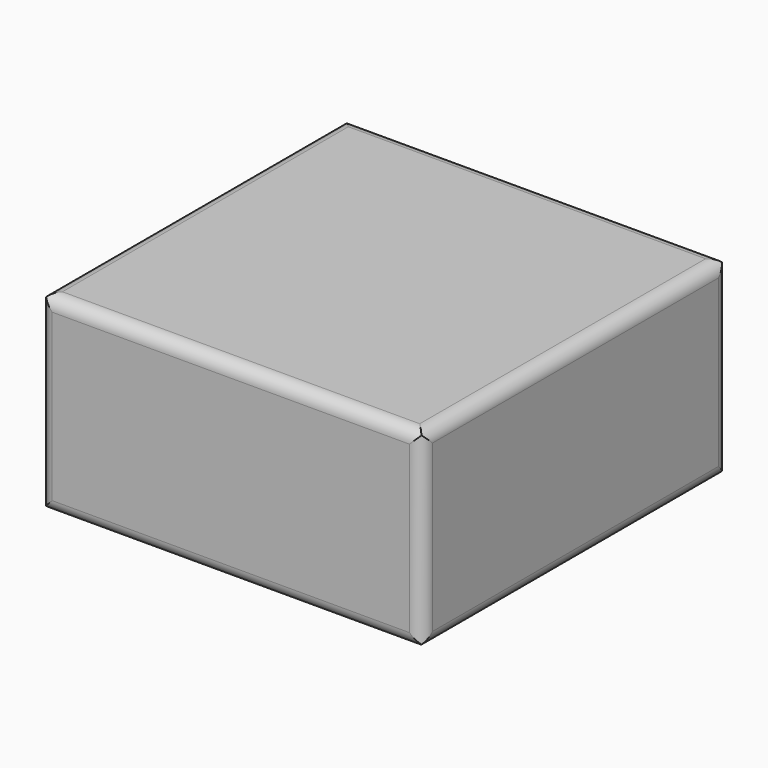
from build123d import *

# Parameters (mm, degrees)
F0_W        = 150
F0_H        = 150
F1_DEPTH    = 75
F2_R        = 5
F3_T1_DEPTH = 170
F3_T3_DEPTH = 100
F4_T1_DEPTH = 170
F4_T3_DEPTH = 100
F5_T1_DEPTH = 165


# Not quite as in the source:
# - a fillet or chamfer that OpenCascade refuses, or shapes differently, is made with other operations: its cross-section is extruded or revolved along the edge and cut away or added


with BuildPart() as f1:
    # F0 (on Top) → F1 (new body)
    with BuildSketch(Plane.XY):
        with Locations((-1.1938624084, 0.1442111853)):
            Rectangle(F0_W, F0_H)
    extrude(amount=F1_DEPTH)

    # F2
    f2_edges = [f1.edges().sort_by_distance(p)[0] for p in [
        (-76.193862, -74.855789, 37.5),
        (73.806138, -74.855789, 37.5),
        (-1.193862, -74.855789, 0),
        (-1.193862, -74.855789, 75),
    ]]
    fillet(f2_edges, radius=F2_R)

    # F3: fillet of radius 5 on 4 edges, made by hand

    # F3_s2 → F3_t1 (cut)
    with BuildSketch(Plane.XZ.offset(-87.6442111853)):
        with BuildLine():
            ThreePointArc((68.8061375916, 0), (72.3416714975, 1.4644660941), (73.8061375916, 5))
            Line((73.8061375916, 5), (73.8061375916, 0))
            Line((73.8061375916, 0), (68.8061375916, 0))
        make_face()
        with BuildLine():
            ThreePointArc((68.8061375916, 75), (72.3416714975, 73.5355339059), (73.8061375916, 70))
            Line((73.8061375916, 70), (73.8061375916, 75))
            Line((73.8061375916, 75), (68.8061375916, 75))
        make_face()
    extrude(amount=F3_T1_DEPTH, mode=Mode.SUBTRACT)

    # F3_s4 → F3_t3 (cut)
    with BuildSketch(Plane.XY.offset(-12.5)):
        with BuildLine():
            ThreePointArc((68.8061375916, 75.1442111853), (72.3416714975, 73.6797450912), (73.8061375916, 70.1442111853))
            Line((73.8061375916, 70.1442111853), (73.8061375916, 75.1442111853))
            Line((73.8061375916, 75.1442111853), (68.8061375916, 75.1442111853))
        make_face()
    extrude(amount=F3_T3_DEPTH, mode=Mode.SUBTRACT)

    # F4: fillet of radius 5 on 4 edges, made by hand

    # F4_s2 → F4_t1 (cut)
    with BuildSketch(Plane.YZ.offset(-88.6938624084)):
        with BuildLine():
            ThreePointArc((70.1442111853, 0), (73.6797450912, 1.4644660941), (75.1442111853, 5))
            Line((75.1442111853, 5), (75.1442111853, 0))
            Line((75.1442111853, 0), (70.1442111853, 0))
        make_face()
        with BuildLine():
            ThreePointArc((75.1442111853, 70), (73.6797450912, 73.5355339059), (70.1442111853, 75))
            Line((70.1442111853, 75), (75.1442111853, 75))
            Line((75.1442111853, 75), (75.1442111853, 70))
        make_face()
    extrude(amount=F4_T1_DEPTH, mode=Mode.SUBTRACT)

    # F4_s4 → F4_t3 (cut)
    with BuildSketch(Plane.XY.offset(-12.5)):
        with BuildLine():
            ThreePointArc((-76.1938624084, 70.1442111853), (-74.7293963143, 73.6797450912), (-71.1938624084, 75.1442111853))
            Line((-71.1938624084, 75.1442111853), (-76.1938624084, 75.1442111853))
            Line((-76.1938624084, 75.1442111853), (-76.1938624084, 70.1442111853))
        make_face()
    extrude(amount=F4_T3_DEPTH, mode=Mode.SUBTRACT)

    # F5: fillet of radius 5 on 4 edges, made by hand

    # F5_s2 → F5_t1 (cut)
    with BuildSketch(Plane.XZ.offset(-82.6442111853)):
        with BuildLine():
            ThreePointArc((-76.1938624084, 5), (-74.7293963143, 1.4644660941), (-71.1938624084, 0))
            Line((-71.1938624084, 0), (-76.1938624084, 0))
            Line((-76.1938624084, 0), (-76.1938624084, 5))
        make_face()
        with BuildLine():
            ThreePointArc((-76.1938624084, 70), (-74.7293963143, 73.5355339059), (-71.1938624084, 75))
            Line((-71.1938624084, 75), (-76.1938624084, 75))
            Line((-76.1938624084, 75), (-76.1938624084, 70))
        make_face()
    extrude(amount=F5_T1_DEPTH, mode=Mode.SUBTRACT)


solid = f1.part
